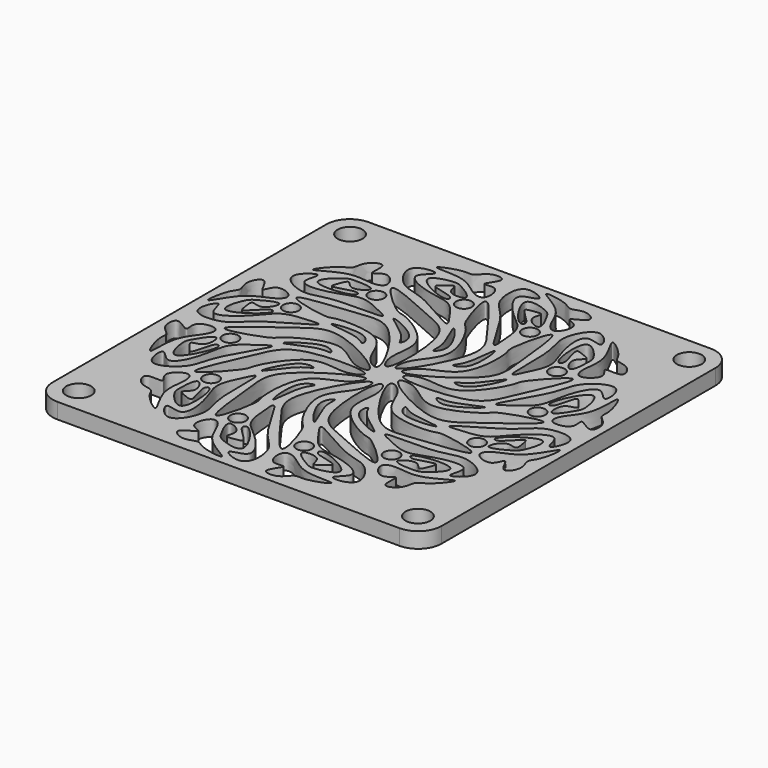
from build123d import *

# Parameters (mm, degrees)
F0_W            = 50
F0_H            = 50
F1_DEPTH        = 2
F2_D            = 3.2
F3_R            = 0.9994506969
F4_DEPTH        = 2.001
F4_COPIES_COUNT = 12
F6_R            = 3


# Not quite as in the source:
# - a pattern or mirror of a feature is missing from the dataset's text; its kind, count and spacing are read off the source's solid
# - a feature names something its author has since deleted; it is built from what else it names


with BuildPart() as f1:
    # F0 (on Top) → F1 (new body)
    with BuildSketch(Plane.XY):
        Rectangle(F0_W, F0_H)
    extrude(amount=F1_DEPTH)

    # F2 (through all)
    with Locations(Plane(origin=(0, 0, 0), x_dir=(1, 0, 0), z_dir=(0, 0, -1))):
        with Locations((-21.8, -21.8), (21.8, -21.8), (21.8, 21.8), (-21.8, 21.8)):
            Hole(F2_D / 2)

    # F3 (on face) → F4 (cut, through all)
    with BuildSketch(Plane.XY.offset(2)):
        with BuildLine():
            add(Edge.make_bspline(
                [(0.0294623442, 1.9401652971), (0.8482367605, 1.9580668147), (5.5191891188, 9.9052471392), (2.5087120543, 13.1588857059), (-3.5931151268, 22.1269956596), (-0.8497216989, 13.550608654), (0.0245187016, 13.5135616868), (3.6110138418, 7.3161075374), (-0.3455475602, 4.4523767198), (-0.3601048278, 1.9316478796), (0.0294623442, 1.9401652971)],
                knots=[0, 0, 0, 0, 0.1677594923, 0.3055536083, 0.4546306649, 0.5859683016, 0.6519419471, 0.7936784485, 0.9201812005, 1, 1, 1, 1], degree=3))
        make_face()
        with BuildLine():
            add(Edge.make_bspline(
                [(4.5303539373, 12.0569951832), (4.1114165601, 12.1070394446), (1.3621892646, 17.9356803167), (-1.4386078661, 19.2281344706), (-1.5544598692, 24.6673017162), (3.1466611175, 22.423385629), (-1.3682403245, 22.3421423546), (1.6670621758, 18.2841905752), (4.3142378961, 16.7633613444), (4.5602724122, 13.9631287959), (4.7464540919, 12.0311808892), (4.5303539373, 12.0569951832)],
                knots=[0, 0, 0, 0, 0.1542022107, 0.2771903297, 0.3946819719, 0.4926408046, 0.5802222419, 0.6993120573, 0.8134230388, 0.9204579887, 1, 1, 1, 1], degree=3))
        make_face()
        with BuildLine():
            add(Edge.make_bspline(
                [(-0.8730257978, 12.2857335955), (-0.6594848957, 12.3430221937), (2.2246497036, 8.6860537226), (0.1573477777, 6.7058748919), (0.9214398646, 8.7084551781), (-1.0778496977, 12.2307835883), (-0.8730257978, 12.2857335955)],
                knots=[0, 0, 0, 0, 0.3179966618, 0.5115036984, 0.6949843528, 1, 1, 1, 1], degree=3))
        make_face()
        with BuildLine():
            add(Edge.make_bspline(
                [(1.1703841155, 21.3084928691), (1.4130051618, 21.9498262522), (4.1254151184, 21.1541755241), (4.7430998121, 20.3901556325), (6.4466209986, 17.034548908), (3.2649433561, 18.6950014152), (4.5604834978, 20.5176985694), (2.9089016666, 20.1716748297), (1.4858169757, 19.9995341299), (4.4295024395, 17.9900668357), (3.5360034078, 16.6283883621), (0.8428205727, 20.4426263734), (1.1703841155, 21.3084928691)],
                knots=[0, 0, 0, 0, 0.1195809755, 0.2124384962, 0.3255250599, 0.4275164574, 0.5138701311, 0.5947479724, 0.6599944061, 0.784025377, 0.838553297, 1, 1, 1, 1], degree=3))
        make_face()
        with BuildLine():
            add(Edge.make_bspline(
                [(4.3760398403, 23.5524531454), (3.4886606707, 23.9230002814), (-0.0700159777, 24.46353327), (5.3384676214, 22.1477424061), (5.8967533306, 18.8963791175), (7.6258114601, 17.6245102839), (8.8923105057, 20.6910090592), (5.9355490573, 21.0630920255), (9.5652569087, 22.1596445637), (7.1371421727, 23.736826515), (5.500897808, 22.6100316698), (5.0057029672, 23.2895217217), (4.3760398403, 23.5524531454)],
                knots=[0, 0, 0, 0, 0.1148597918, 0.2443981151, 0.3767478509, 0.4568007914, 0.5599087242, 0.6419074154, 0.7384926058, 0.8277971733, 0.918498227, 1, 1, 1, 1], degree=3))
        make_face()
        with Locations((5.6048748083, 16.4465811104)):
            Circle(F3_R)
    f4 = extrude(amount=-F4_DEPTH, mode=Mode.SUBTRACT)

    # F4_copies: F4 ×12 about axis
    f4_copies_axis = Axis((0, 0, 0), (0, 0, 1))
    for i in range(1, F4_COPIES_COUNT):
        add(f4.rotate(f4_copies_axis, i * 360 / F4_COPIES_COUNT), mode=Mode.SUBTRACT)

    # F6
    f6_edges = [f1.edges().sort_by_distance(p)[0] for p in [
        (-25, 25, 1),
        (25, 25, 1),
        (25, -25, 1),
        (-25, -25, 1),
    ]]
    fillet(f6_edges, radius=F6_R)


solid = f1.part
